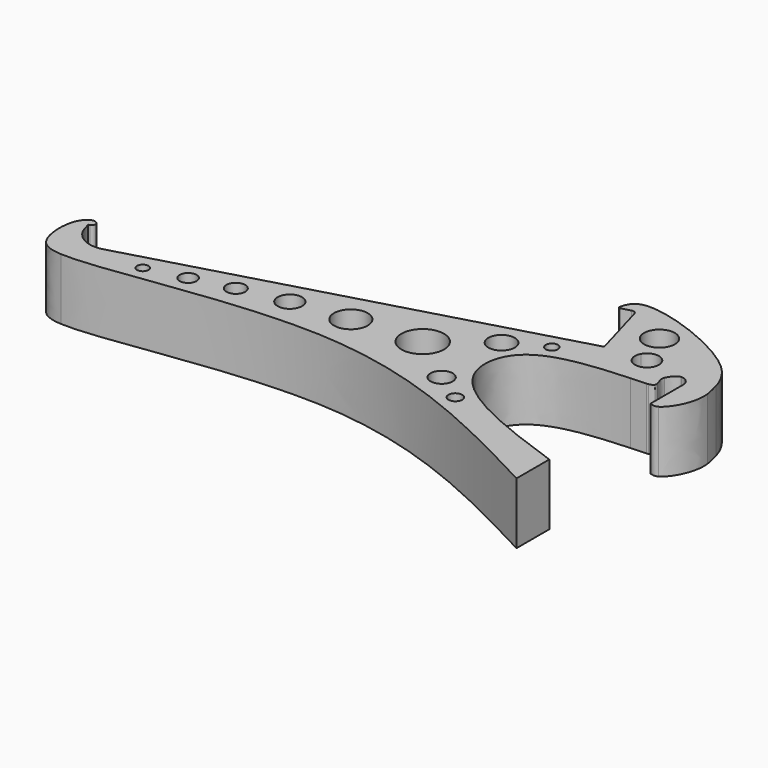
from build123d import *

# Parameters (mm, degrees)
F0_R     = 1.7576231228
F0_R_2   = 2.6194646955
F0_R_3   = 2.9064395042
F0_R_4   = 3.7846862671
F0_R_5   = 5.2290610065
F0_R_6   = 2.1208004667
F0_R_7   = 3.4250228461
F0_R_8   = 6.5999331713
F0_R_9   = 4.0939669446
F0_R_10  = 1.8790687222
F1_DEPTH = 19.05
F2_R     = 8.382
F3_R     = 1.27
F4_R     = 0.508
F5_R     = 2.54
F6_R     = 1.143


# Not quite as in the source:
# - a feature names something its author has since deleted; it is built from what else it names


with BuildPart() as f1:
    # F0 (on Top) → F1 (new body)
    with BuildSketch(Plane.XY):
        with BuildLine():
            Line((10.541, 0), (2.921, 0))
            Line((2.921, 0), (2.921, -10.128200235))
            ThreePointArc((2.921, -10.128200235), (5.467200091, -9.0123473171), (7.633137931, -7.2696551724))
            Line((7.633137931, -7.2696551724), (10.541, 0))
        make_face()
        with BuildLine():
            ThreePointArc((0, 2.921), (2.0654589078, 2.0654589078), (2.921, 0))
            Line((2.921, 0), (10.541, 0))
            add(Edge.make_bspline(
                [(9.4647116957, 4.6402492947), (9.9365749021, 3.093212593), (10.238787451, 1.5466062965), (10.541, 0)],
                knots=[0.8946694577, 0.8946694577, 0.8946694577, 0.8946694577, 1, 1, 1, 1], degree=3))
            ThreePointArc((9.4647116957, 4.6402492947), (5.5767290227, 8.9449859926), (0, 10.541))
            Line((0, 10.541), (0, 2.921))
        make_face()
        with BuildLine():
            add(Edge.make_bspline(
                [(-2.3848635838, -3.2166666053), (-2.4728326484, -2.8639169674), (-2.9207971155, -1.7035058727), (-3.2431227864, -0.8639813892), (-2.921, 0)],
                knots=[0.2535057974, 0.2535057974, 0.2535057974, 0.2535057974, 0.3356664829, 0.509164944, 0.509164944, 0.509164944, 0.509164944], degree=3))
            ThreePointArc((-2.921, 0), (-2.0933427309, 2.0371934643), (-0.0793997186, 2.9199206641))
            add(Edge.make_bspline(
                [(-0.0793997186, 2.9199206641), (-0.0526154408, 2.921489703), (-0.0261396552, 2.9218637368), (0, 2.921)],
                knots=[0.7428905608, 0.7428905608, 0.7428905608, 0.7428905608, 0.749200115, 0.749200115, 0.749200115, 0.749200115], degree=3))
            Line((0, 2.921), (0, 10.541))
            Line((0, 10.541), (-5.5241232696, 8.977568886))
            ThreePointArc((-5.5241232696, 8.977568886), (-7.185645683, 7.7122744453), (-8.5651021417, 6.1442417191))
            ThreePointArc((-8.5651021417, 6.1442417191), (-8.2751102539, 5.3401365451), (-8.1767075611, 4.4910209253))
            ThreePointArc((-8.1767075611, 4.4910209253), (-8.8083299958, 2.4195216624), (-10.4882883034, 1.0528482629))
            ThreePointArc((-10.4882883034, 1.0528482629), (-10.3010896952, -2.2361198743), (-9.1077855872, -5.3066866025))
            add(Edge.make_bspline(
                [(-9.1077855872, -5.3066866025), (-7.4549936416, -5.2237610648), (-5.7884221322, -5.1507653072), (-4.1215360581, -5.0777890942)],
                knots=[0.9571200697, 0.9571200697, 0.9571200697, 0.9571200697, 1, 1, 1, 1], degree=3))
            add(Edge.make_bspline(
                [(-4.1215360581, -5.0777890942), (-3.3682495324, -4.8980809941), (-2.6149630067, -4.7183728941), (-2.3848635838, -4.2266139709)],
                knots=[0, 0, 0, 0, 0.1642422553, 0.1642422553, 0.1642422553, 0.1642422553], degree=3))
            Line((-2.3848635838, -4.2266139709), (-2.3848635838, -3.2166666053))
        make_face()
        with BuildLine():
            ThreePointArc((-0.0793997186, 2.9199206641), (-2.0933427309, 2.0371934643), (-2.921, 0))
            add(Edge.make_bspline(
                [(-2.921, 0), (-2.4870575516, 1.1638984113), (-1.0715731361, 2.8617985559), (-0.0793997186, 2.9199206641)],
                knots=[0.509164944, 0.509164944, 0.509164944, 0.509164944, 0.7428905608, 0.7428905608, 0.7428905608, 0.7428905608], degree=3))
        make_face()
        with BuildLine():
            add(Edge.make_bspline(
                [(-2.3848635838, -4.2266139709), (-2.2598075227, -3.9593493547), (-2.2892895236, -3.5999117297), (-2.3848635838, -3.2166666053)],
                knots=[0.1642422553, 0.1642422553, 0.1642422553, 0.1642422553, 0.2535057974, 0.2535057974, 0.2535057974, 0.2535057974], degree=3))
            Line((-2.3848635838, -3.2166666053), (-2.3848635838, -4.2266139709))
        make_face()
        with BuildLine():
            ThreePointArc((7.633137931, -7.2696551724), (5.467200091, -9.0123473171), (2.921, -10.128200235))
            Line((2.921, -10.128200235), (2.921, -12.7))
            Line((2.921, -12.7), (5.461, -12.7))
            Line((5.461, -12.7), (7.633137931, -7.2696551724))
        make_face()
        with BuildLine():
            ThreePointArc((7.633137931, -7.2696551724), (9.7870727986, -3.9148291194), (10.541, 0))
            Line((10.541, 0), (7.633137931, -7.2696551724))
        make_face()
        with BuildLine():
            add(Edge.make_bspline(
                [(10.541, 0), (11.2509652972, -5.7718935423), (7.6916234008, -11.4340619195), (5.461, -12.7)],
                knots=[0, 0, 0, 0, 0.6988492234, 0.6988492234, 0.6988492234, 0.6988492234], degree=3))
            ThreePointArc((10.541, 0), (9.7870727986, -3.9148291194), (7.633137931, -7.2696551724))
            Line((7.633137931, -7.2696551724), (5.461, -12.7))
        make_face()
        with BuildLine():
            Line((-16.6670959443, 10.541), (0, 10.541))
            ThreePointArc((0, 10.541), (5.5767290227, 8.9449859926), (9.4647116957, 4.6402492947))
            add(Edge.make_bspline(
                [(-30.9420047574, 26.5976409188), (-24.3766956681, 28.1974465791), (3.1561278341, 17.9494181138), (8.5138708016, 7.7576480258), (9.4647116957, 4.6402492947)],
                knots=[0.2011479798, 0.2011479798, 0.2011479798, 0.2011479798, 0.6824202598, 0.8946694577, 0.8946694577, 0.8946694577, 0.8946694577], degree=3))
            Line((-30.9420047574, 26.5976409188), (-29.9044561627, 22.9316358842))
            Line((-29.9044561627, 22.9316358842), (-26.3976724219, 10.541))
            Line((-26.3976724219, 10.541), (-16.6670959443, 10.541))
        make_face()
        with BuildLine():
            ThreePointArc((-11.9050923426, 15.3030036017), (-13.2998509055, 11.9357585629), (-16.6670959443, 10.541))
            ThreePointArc((-16.6670959443, 10.541), (-20.0343409831, 18.6702486405), (-11.9050923426, 15.3030036017))
        make_face(mode=Mode.SUBTRACT)
        with BuildLine():
            Line((-5.5241232696, 8.977568886), (0, 10.541))
            ThreePointArc((0, 10.541), (-2.870551112, 10.142613929), (-5.5241232696, 8.977568886))
        make_face()
        with BuildLine():
            ThreePointArc((-5.5241232696, 8.977568886), (-2.870551112, 10.142613929), (0, 10.541))
            Line((0, 10.541), (-16.6670959443, 10.541))
            Line((-16.6670959443, 10.541), (-26.3976724219, 10.541))
            Line((-26.3976724219, 10.541), (-24.4400335639, 3.6240093687))
            Line((-24.4400335639, 3.6240093687), (-15.1585403449, 6.2508470722))
            ThreePointArc((-15.1585403449, 6.2508470722), (-12.9004660988, 8.0634085442), (-10.0274151455, 7.7030523173))
            Line((-10.0274151455, 7.7030523173), (-5.5241232696, 8.977568886))
        make_face()
        with BuildLine():
            Line((5.461, -12.7), (2.921, -12.7))
            add(Edge.make_bspline(
                [(5.461, -12.7), (4.4997712444, -13.2455228729), (3.7852793191, -12.9746862741), (2.921, -12.7)],
                knots=[0.6988492234, 0.6988492234, 0.6988492234, 0.6988492234, 1, 1, 1, 1], degree=3))
        make_face()
        with BuildLine():
            add(Edge.make_bspline(
                [(2.0828, -50.8), (-15.8735350331, -44.4526794588), (-44.1502352976, -34.2737591947), (-40.756956224, -7.8620336461), (-20.8847334133, -5.8975714593), (-9.1077855872, -5.3066866025)],
                knots=[0, 0, 0, 0, 0.408994296, 0.651579676, 0.9571200697, 0.9571200697, 0.9571200697, 0.9571200697], degree=3))
            ThreePointArc((-9.1077855872, -5.3066866025), (-10.3010896952, -2.2361198743), (-10.4882883034, 1.0528482629))
            ThreePointArc((-10.4882883034, 1.0528482629), (-14.6511436849, 2.009685541), (-15.1585403449, 6.2508470722))
            Line((-15.1585403449, 6.2508470722), (-24.4400335639, 3.6240093687))
            Line((-24.4400335639, 3.6240093687), (-38.5809545016, -0.3781380665))
            Line((-38.5809545016, -0.3781380665), (-134.62, -27.559))
            Line((-134.62, -27.559), (-159.0600335639, -34.4759906313))
            Line((-159.0600335639, -34.4759906313), (-157.3307859061, -40.5859990223))
            add(Edge.make_bspline(
                [(-157.3307859061, -40.5859990223), (-144.0553777211, -41.3698511276), (-73.62744163, -23.7523445291), (-24.481821439, -49.5498829603), (2.0828, -63.5)],
                knots=[0.3634781173, 0.3634781173, 0.3634781173, 0.3634781173, 0.6705750285, 1, 1, 1, 1], degree=3))
            Line((2.0828, -63.5), (2.0828, -50.8))
        make_face()
        with Locations((-137.4377459288, -33.8753685355)):
            Circle(F0_R, mode=Mode.SUBTRACT)
        with Locations((-125.5742162466, -31.133711338)):
            Circle(F0_R_2, mode=Mode.SUBTRACT)
        with Locations((-113.1754145026, -28.1649827957)):
            Circle(F0_R_3, mode=Mode.SUBTRACT)
        with Locations((-98.6075103283, -25.4469309002)):
            Circle(F0_R_4, mode=Mode.SUBTRACT)
        with Locations((-81.2796056271, -23.4645009041)):
            Circle(F0_R_5, mode=Mode.SUBTRACT)
        with Locations((-36.0271334648, -39.5576246083)):
            Circle(F0_R_6, mode=Mode.SUBTRACT)
        with Locations((-45.155338943, -33.4500707686)):
            Circle(F0_R_7, mode=Mode.SUBTRACT)
        with Locations((-60.4273863137, -21.702343598)):
            Circle(F0_R_8, mode=Mode.SUBTRACT)
        with Locations((-45.155338943, -10.2483071387)):
            Circle(F0_R_9, mode=Mode.SUBTRACT)
        with Locations((-34.2323705554, -4.4191675261)):
            Circle(F0_R_10, mode=Mode.SUBTRACT)
        with BuildLine():
            ThreePointArc((-8.5651021417, 6.1442417191), (-7.185645683, 7.7122744453), (-5.5241232696, 8.977568886))
            Line((-5.5241232696, 8.977568886), (-10.0274151455, 7.7030523173))
            ThreePointArc((-10.0274151455, 7.7030523173), (-9.1816607704, 7.0311507523), (-8.5651021417, 6.1442417191))
        make_face()
        with BuildLine():
            Line((-29.9044561627, 22.9316358842), (-30.9420047574, 26.5976409188))
            add(Edge.make_bspline(
                [(-34.7924628755, 21.5482377579), (-34.2392208548, 23.7386195676), (-33.6859788341, 25.9290013773), (-30.9420047574, 26.5976409188)],
                knots=[0, 0, 0, 0, 0.2011479798, 0.2011479798, 0.2011479798, 0.2011479798], degree=3))
            Line((-34.7924628755, 21.5482377579), (-29.9044561627, 22.9316358842))
        make_face()
        with BuildLine():
            add(Edge.make_bspline(
                [(-165.1700419549, -36.2052382891), (-163.9966596031, -38.9594916297), (-161.8785228938, -40.3174759635), (-157.3307859061, -40.5859990223)],
                knots=[0.2582763817, 0.2582763817, 0.2582763817, 0.2582763817, 0.3634781173, 0.3634781173, 0.3634781173, 0.3634781173], degree=3))
            Line((-157.3307859061, -40.5859990223), (-159.0600335639, -34.4759906313))
            Line((-159.0600335639, -34.4759906313), (-165.1700419549, -36.2052382891))
        make_face()
        with BuildLine():
            Line((-165.1700419549, -36.2052382891), (-159.0600335639, -34.4759906313))
            Line((-159.0600335639, -34.4759906313), (-161.8959997228, -24.4555768701))
            Line((-161.8959997228, -24.4555768701), (-165.5620047574, -25.4931254648))
            add(Edge.make_bspline(
                [(-165.5620047574, -25.4931254648), (-166.6062770263, -28.5203024248), (-166.4520124462, -33.1960985126), (-165.1700419549, -36.2052382891)],
                knots=[0.1433389784, 0.1433389784, 0.1433389784, 0.1433389784, 0.2582763817, 0.2582763817, 0.2582763817, 0.2582763817], degree=3))
        make_face()
        with BuildLine():
            Line((-162.5876987859, -22.0115735137), (-161.8959997228, -24.4555768701))
            Line((-161.8959997228, -24.4555768701), (-159.2075960307, -23.6947079006))
            add(Edge.make_bspline(
                [(-159.2075960307, -23.6947079006), (-160.6750664221, -22.4582941647), (-161.5912860772, -21.8038515678), (-162.5876987859, -22.0115735137)],
                knots=[0, 0, 0, 0, 0.0682171341, 0.0682171341, 0.0682171341, 0.0682171341], degree=3))
        make_face()
        with BuildLine():
            Line((-165.5620047574, -25.4931254648), (-161.8959997228, -24.4555768701))
            Line((-161.8959997228, -24.4555768701), (-162.5876987859, -22.0115735137))
            add(Edge.make_bspline(
                [(-162.5876987859, -22.0115735137), (-163.6849650577, -22.2403203804), (-164.8794796913, -23.5145953285), (-165.5620047574, -25.4931254648)],
                knots=[0.0682171341, 0.0682171341, 0.0682171341, 0.0682171341, 0.1433389784, 0.1433389784, 0.1433389784, 0.1433389784], degree=3))
        make_face()
    extrude(amount=F1_DEPTH)

    # F2
    f2_edges = [f1.edges().sort_by_distance(p)[0] for p in [
        (-159.060034, -34.475991, 9.525),
    ]]
    fillet(f2_edges, radius=F2_R)

    # F3
    f3_edges = [f1.edges().sort_by_distance(p)[0] for p in [
        (-29.904456, 22.931636, 9.525),
    ]]
    fillet(f3_edges, radius=F3_R)

    # F4
    f4_edges = [f1.edges().sort_by_distance(p)[0] for p in [
        (-34.792463, 21.548238, 9.525),
    ]]
    fillet(f4_edges, radius=F4_R)

    # F5
    f5_edges = [f1.edges().sort_by_distance(p)[0] for p in [
        (-4.121536, -5.077789, 9.525),
    ]]
    fillet(f5_edges, radius=F5_R)

    # F6
    f6_edges = [f1.edges().sort_by_distance(p)[0] for p in [
        (-159.207596, -23.694708, 9.525),
    ]]
    fillet(f6_edges, radius=F6_R)


solid = f1.part
